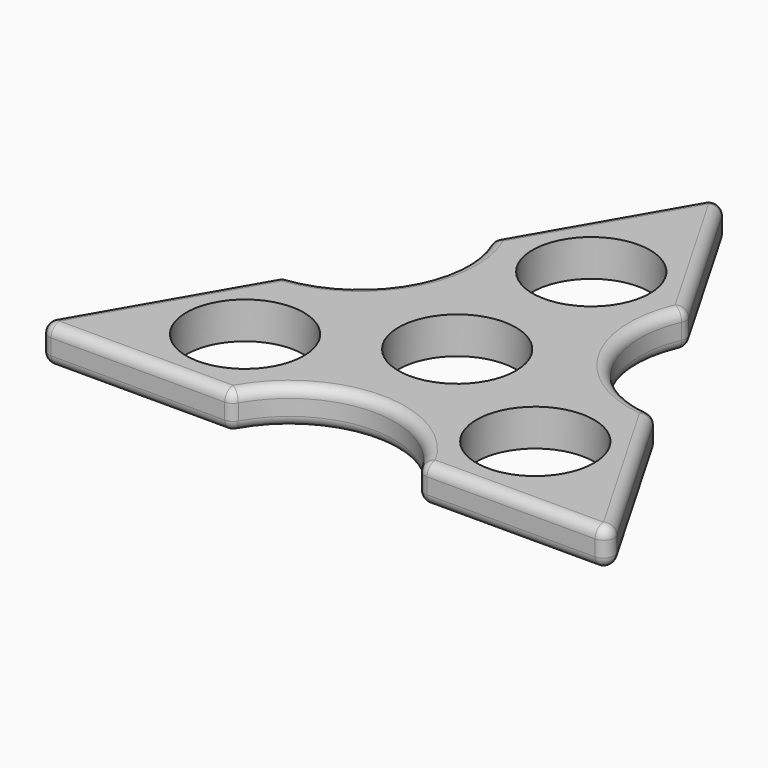
from build123d import *

# Parameters (mm, degrees)
F0_R     = 11.15
F1_DEPTH = 7
F2_R     = 2


# Not quite as in the source:
# - a feature names something its author has since deleted; it is built from what else it names


with BuildPart() as f1:
    # F0 (on Top) → F1 (new body)
    with BuildSketch(Plane.XY):
        with BuildLine():
            Line((18.6057756776, 31.4331508418), (0, 63.6592996296))
            Line((0, 63.6592996296), (-18.6057756776, 31.4331508418))
            ThreePointArc((-18.6057756776, 31.4331508418), (-19.2524106529, 12.6478352194), (-35.1976537124, 2.6951750926))
            Line((-35.1976537124, 2.6951750926), (-55.1305706664, -31.8296498148))
            Line((-55.1305706664, -31.8296498148), (-17.4760334194, -31.8296498148))
            ThreePointArc((-17.4760334194, -31.8296498148), (0.5244189685, -20.546513576), (18.5248713564, -31.8296498148))
            Line((18.5248713564, -31.8296498148), (55.1305706664, -31.8296498148))
            Line((55.1305706664, -31.8296498148), (35.1976537124, 2.6951750926))
            ThreePointArc((35.1976537124, 2.6951750926), (19.2524106529, 12.6478352194), (18.6057756776, 31.4331508418))
        make_face()
        with Locations((-27.5652853332, -15.9148249074)):
            Circle(F0_R, mode=Mode.SUBTRACT)
        with Locations((27.5652853332, -15.9148249074)):
            Circle(F0_R, mode=Mode.SUBTRACT)
        Circle(F0_R, mode=Mode.SUBTRACT)
        with Locations((0, 31.8296498148)):
            Circle(F0_R, mode=Mode.SUBTRACT)
    extrude(amount=F1_DEPTH)

    # F2
    f2_edges = [f1.edges().sort_by_distance(p)[0] for p in [
        (55.130571, -31.82965, 3.5),
        (35.197654, 2.695175, 3.5),
        (45.164112, -14.567237, 0),
        (45.164112, -14.567237, 7),
        (18.605776, 31.433151, 3.5),
        (19.252411, 12.647835, 0),
        (19.252411, 12.647835, 7),
        (0, 63.6593, 3.5),
        (9.302888, 47.546225, 0),
        (9.302888, 47.546225, 7),
        (-18.605776, 31.433151, 3.5),
        (-9.302888, 47.546225, 0),
        (-9.302888, 47.546225, 7),
        (-35.197654, 2.695175, 3.5),
        (-19.252411, 12.647835, 0),
        (-19.252411, 12.647835, 7),
        (-55.130571, -31.82965, 3.5),
        (-45.164112, -14.567237, 0),
        (-45.164112, -14.567237, 7),
        (-17.476033, -31.82965, 3.5),
        (18.524871, -31.82965, 3.5),
        (0.524419, -20.546514, 0),
        (0.524419, -20.546514, 7),
        (-36.303302, -31.82965, 0),
        (-36.303302, -31.82965, 7),
        (36.827721, -31.82965, 0),
        (36.827721, -31.82965, 7),
    ]]
    fillet(f2_edges, radius=F2_R)


solid = f1.part
